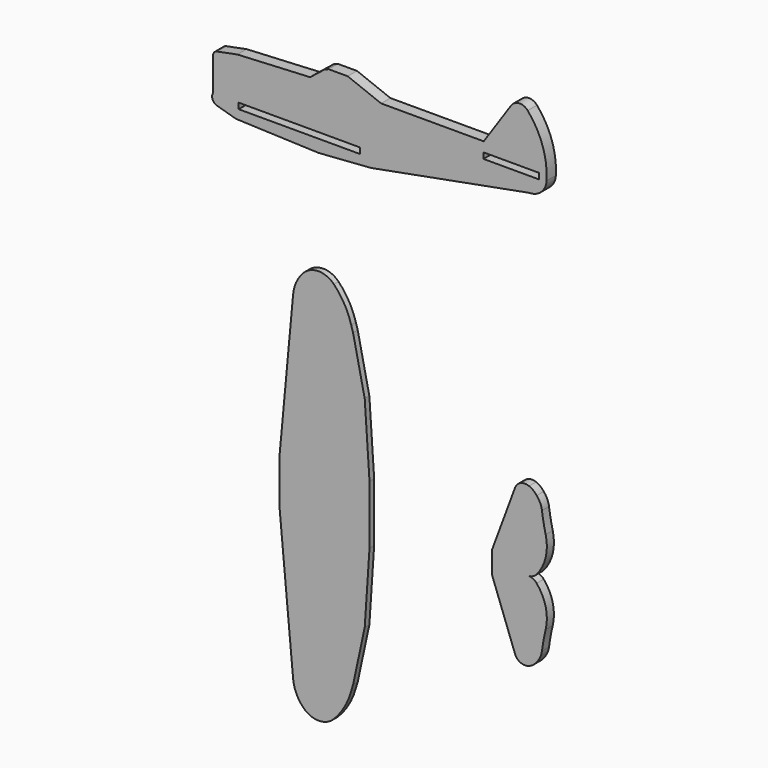
from build123d import *

# Parameters (mm, degrees)
F2_DEPTH = 3.175
F3_DEPTH = 3.175
F4_W     = 66.3537942724
F4_H     = 3.175
F4_W_2   = 30.48
F5_DEPTH = 6.351
F6_DEPTH = 1.651


# Not quite as in the source:
# - a length typed as a fraction of an inch, garbled in the dataset ("3 / 203.2 mm" for 3/8 in), is restored


with BuildPart() as f2:
    # F1 (on Front) → F2 (new body)
    with BuildSketch(Plane.XZ):
        with BuildLine():
            Line((-172.6110667898, 206.8775344049), (-179.9945831299, 127.231195569))
            Line((-179.9945831299, 127.231195569), (-179.9945831299, 114.4247949123))
            Line((-179.9945831299, 114.4247949123), (-179.9945831299, 101.6183942556))
            Line((-179.9945831299, 101.6183942556), (-172.6110667898, 21.9720554197))
            ThreePointArc((-172.6110667898, 21.9720554197), (-170.845271575, 15.3895933308), (-166.9893544961, 9.7700966119))
            ThreePointArc((-166.9893544961, 9.7700966119), (-158.643886447, 6.2428365844), (-150.2984183978, 9.7700966119))
            ThreePointArc((-150.2984183978, 9.7700966119), (-144.5228447898, 17.4405844589), (-140.8358120402, 26.3062160673))
            ThreePointArc((-140.8358120402, 26.3062160673), (-140.3408665737, 28.0234348127), (-139.8043911336, 29.7281357651))
            Line((-139.8043911336, 29.7281357651), (-133.4421634674, 59.3172758818))
            Line((-133.4421634674, 59.3172758818), (-130.8142542839, 98.4076410532))
            Line((-130.8142542839, 98.4076410532), (-130.8142542839, 114.4247949123))
            Line((-130.8142542839, 114.4247949123), (-130.8142542839, 130.4419487715))
            Line((-130.8142542839, 130.4419487715), (-133.4421634674, 169.5323139429))
            Line((-133.4421634674, 169.5323139429), (-139.8043911336, 199.1214540596))
            ThreePointArc((-139.8043911336, 199.1214540596), (-140.3408665737, 200.8261550119), (-140.8358120402, 202.5433737574))
            ThreePointArc((-140.8358120402, 202.5433737574), (-144.5228447898, 211.4090053658), (-150.2984183978, 219.0794932127))
            ThreePointArc((-150.2984183978, 219.0794932127), (-158.643886447, 222.6067532402), (-166.9893544961, 219.0794932127))
            ThreePointArc((-166.9893544961, 219.0794932127), (-170.845271575, 213.4599964938), (-172.6110667898, 206.8775344049))
        make_face()
    extrude(amount=F2_DEPTH)


with BuildPart() as f2b:
    # F1 (on Front) → F2, piece 2 (new body)
    with BuildSketch(Plane.XZ):
        with BuildLine():
            Line((-213.8443440199, 309.9319636822), (-213.8443440199, 291.8651401997))
            ThreePointArc((-213.8443440199, 291.8651401997), (-214.1212611685, 288.6056865576), (-211.7022424936, 286.4036262035))
            Line((-211.7022424936, 286.4036262035), (-201.2821733952, 283.4078669548))
            Line((-201.2821733952, 283.4078669548), (-156.0851335526, 281.714618206))
            Line((-156.0851335526, 281.714618206), (-127.429947257, 283.798635006))
            Line((-127.429947257, 283.798635006), (-40.9433990717, 299.9497354031))
            ThreePointArc((-40.9433990717, 299.9497354031), (-34.41478075, 302.4733352076), (-31.4350910485, 308.8068068027))
            ThreePointArc((-31.4350910485, 308.8068068027), (-33.6156920244, 325.0469200325), (-41.7249053717, 339.285492897))
            ThreePointArc((-41.7249053717, 339.285492897), (-46.4124339616, 341.278099702), (-50.8424639702, 338.7644886971))
            Line((-50.8424639702, 338.7644886971), (-65.8213049173, 316.6650235653))
            Line((-65.8213049173, 316.6650235653), (-121.9594106078, 316.6650235653))
            Line((-121.9594106078, 316.6650235653), (-140.1952803135, 323.8029181957))
            Line((-140.1952803135, 323.8029181957), (-150.6517082453, 323.8029181957))
            Line((-150.6517082453, 323.8029181957), (-152.9593467712, 322.8657543659))
            Line((-152.9593467712, 322.8657543659), (-160.7475876808, 316.6650235653))
            Line((-160.7475876808, 316.6650235653), (-200.554177165, 314.651042223))
            Line((-200.554177165, 314.651042223), (-211.5154117346, 312.4890625477))
            ThreePointArc((-211.5154117346, 312.4890625477), (-213.174849499, 311.6613190677), (-213.8443440199, 309.9319636822))
        make_face()
    extrude(amount=F2_DEPTH)

    # F3 (add): a face of the model
    f3_faces = [f2b.faces().sort_by_distance(p)[0] for p in [
        (-124.5842443217, -3.175, 304.2983822932),
    ]]
    extrude(f3_faces, amount=F3_DEPTH)

    # F4 (on Front) → F5 (cut, through all)
    with BuildSketch(Plane.XZ):
        with Locations((-166.6496883212, 290.1289781431)):
            Rectangle(F4_W, F4_H)
        with Locations((-50.7230447626, 309.7342949867)):
            Rectangle(F4_W_2, F4_H)
    extrude(amount=F5_DEPTH, mode=Mode.SUBTRACT)


with BuildPart() as f2c:
    # F1 (on Front) → F2, piece 3 (new body)
    with BuildSketch(Plane.XZ):
        with BuildLine():
            Line((-62.5618458308, 120.2978070905), (-62.5618458308, 114.4247949123))
            Line((-62.5618458308, 114.4247949123), (-62.5618458308, 108.5517827342))
            Line((-62.5618458308, 108.5517827342), (-49.8851687327, 74.3610709906))
            ThreePointArc((-49.8851687327, 74.3610709906), (-48.6307450368, 72.3918746751), (-46.6768778861, 71.1137056351))
            ThreePointArc((-46.6768778861, 71.1137056351), (-44.4525964558, 70.7007257405), (-42.2283150256, 71.1137056351))
            ThreePointArc((-42.2283150256, 71.1137056351), (-39.9097876721, 72.4272505107), (-38.0764007568, 74.3610709906))
            ThreePointArc((-38.0764007568, 74.3610709906), (-36.150795106, 77.2653168267), (-35.1798926376, 80.6119493724))
            ThreePointArc((-35.1798926376, 80.6119493724), (-34.3068965337, 86.1265511206), (-33.1462513848, 91.5878565943))
            ThreePointArc((-33.1462513848, 91.5878565943), (-33.1381821173, 102.5132721235), (-38.0764007568, 112.2589771398))
            ThreePointArc((-38.0764007568, 112.2589771398), (-40.0329250575, 113.7901835089), (-42.4349759833, 114.4247949123))
            ThreePointArc((-42.4349759833, 114.4247949123), (-40.0329250575, 115.0594063158), (-38.0764007568, 116.5906126849))
            ThreePointArc((-38.0764007568, 116.5906126849), (-33.1381821173, 126.3363177012), (-33.1462513848, 137.2617332304))
            ThreePointArc((-33.1462513848, 137.2617332304), (-34.3068965337, 142.7230387041), (-35.1798926376, 148.2376404523))
            ThreePointArc((-35.1798926376, 148.2376404523), (-36.150795106, 151.584272998), (-38.0764007568, 154.4885188341))
            ThreePointArc((-38.0764007568, 154.4885188341), (-39.9097876721, 156.4223393139), (-42.2283150256, 157.7358841896))
            ThreePointArc((-42.2283150256, 157.7358841896), (-44.4525964558, 158.1488640842), (-46.6768778861, 157.7358841896))
            ThreePointArc((-46.6768778861, 157.7358841896), (-48.6307450368, 156.4577151496), (-49.8851687327, 154.4885188341))
            Line((-49.8851687327, 154.4885188341), (-62.5618458308, 120.2978070905))
        make_face()
    extrude(amount=F2_DEPTH)

    # F6 (add): a face of the model
    f6_faces = [f2c.faces().sort_by_distance(p)[0] for p in [
        (-46.1187241122, -3.175, 114.4247949123),
    ]]
    extrude(f6_faces, amount=F6_DEPTH)


solid = Compound([f2.part, f2b.part, f2c.part])
